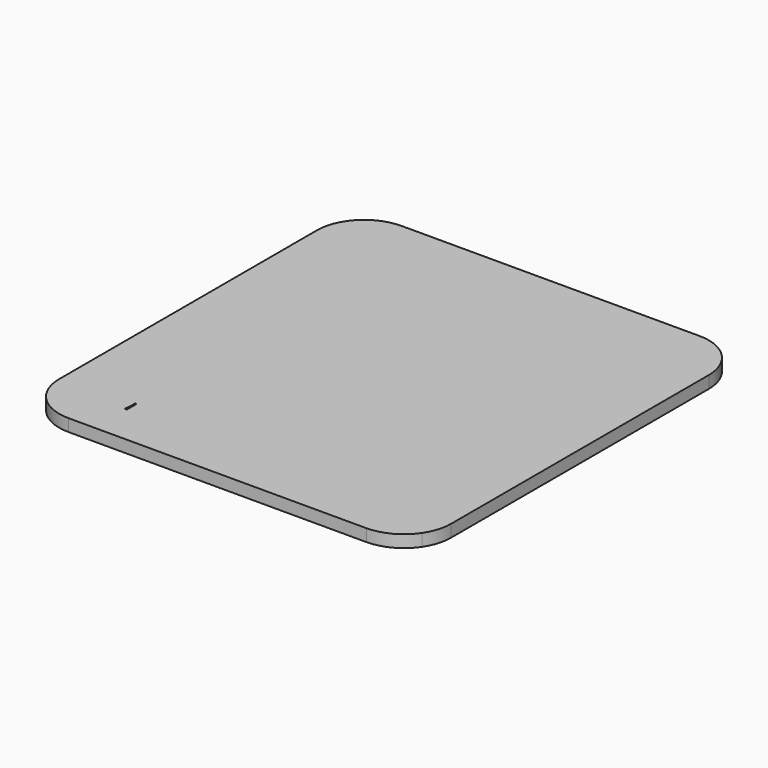
from build123d import *

# Parameters (mm, degrees)
F1_DEPTH = 2
F2_DEPTH = 2
F4_W     = 38
F4_H     = 4
F4_W_2   = 10
F5_DEPTH = 3


# Not quite as in the source:
# - a feature names something its author has since deleted; it is built from what else it names


with BuildPart() as f1:
    # F0 (on Top) → F1 (new body)
    with BuildSketch(Plane.XY):
        with BuildLine():
            Line((24.3022678875, 34), (-24.3022678875, 34))
            ThreePointArc((-24.3022678875, 34), (-29.745386464, 31.745386464), (-32, 26.3022678875))
            Line((-32, 26.3022678875), (-32, 15.1276998222))
            Line((-32, 15.1276998222), (-30.5, 15.1276998222))
            Line((-30.5, 15.1276998222), (-30.5, 21.3020170704))
            Line((-30.5, 21.3020170704), (30.5, 21.3020170704))
            Line((30.5, 21.3020170704), (30.5, 14.2477769405))
            Line((30.5, 14.2477769405), (32, 14.2477769405))
            Line((32, 14.2477769405), (32, 26.3022678875))
            ThreePointArc((32, 26.3022678875), (29.745386464, 31.745386464), (24.3022678875, 34))
        make_face()
        with BuildLine():
            Line((-30.5, 15.1276998222), (-32, 15.1276998222))
            Line((-32, 15.1276998222), (-32, -26.3022678875))
            ThreePointArc((-32, -26.3022678875), (-29.745386464, -31.745386464), (-24.3022678875, -34))
            Line((-24.3022678875, -34), (0, -34))
            Line((0, -34), (24.3022678875, -34))
            ThreePointArc((24.3022678875, -34), (27.9138443036, -33.100178998), (30.6810753302, -30.6110838832))
            ThreePointArc((30.6810753302, -30.6110838832), (31.6628871063, -28.555346757), (32, -26.3022678875))
            Line((32, -26.3022678875), (32, 14.2477769405))
            Line((32, 14.2477769405), (30.5, 14.2477769405))
            Line((30.5, 14.2477769405), (30.5, -14.6979829296))
            Line((30.5, -14.6979829296), (-30.5, -14.6979829296))
            Line((-30.5, -14.6979829296), (-30.5, 15.1276998222))
        make_face()
        with BuildLine():
            ThreePointArc((-20.3994758379, -27.4899639189), (-30.2031719041, -25.7844938681), (-20.255592559, -25.5261339915))
            Line((-20.255592559, -25.5261339915), (-20, -25.5261339915))
            Line((-20, -25.5261339915), (-20, -27.4899639189))
            Line((-20, -27.4899639189), (-20.3994758379, -27.4899639189))
        make_face(mode=Mode.SUBTRACT)
        with BuildLine():
            ThreePointArc((20.2726339823, -25.4029799253), (25.5910239568, -21.1638916046), (30.2165381279, -26.1498479185))
            ThreePointArc((30.2165381279, -26.1498479185), (25.7296627026, -31.1234485429), (20.3218568596, -27.1706786007))
            ThreePointArc((20.3218568596, -27.1706786007), (20.2184754644, -26.2890226707), (20.2726339823, -25.4029799253))
        make_face(mode=Mode.SUBTRACT)
        Polygon((-30.5, 21.3020170704), (-30.5, 15.1276998222), (-30.5, -14.6979829296), (30.5, -14.6979829296), (30.5, 14.2477769405), (30.5, 21.3020170704), align=None)
    extrude(amount=F1_DEPTH)

    # F0 (on Top) → F2 (join)
    with BuildSketch(Plane.XY):
        with BuildLine():
            ThreePointArc((-20.3994758379, -27.4899639189), (-20.2624836545, -26.8261202565), (-20.2165381279, -26.1498479185))
            ThreePointArc((-20.2165381279, -26.1498479185), (-20.2263112871, -25.8373801956), (-20.255592559, -25.5261339915))
            ThreePointArc((-20.255592559, -25.5261339915), (-30.2031719041, -25.7844938681), (-20.3994758379, -27.4899639189))
        make_face()
        with BuildLine():
            ThreePointArc((20.3218568596, -27.1706786007), (25.7296627026, -31.1234485429), (30.2165381279, -26.1498479185))
            ThreePointArc((30.2165381279, -26.1498479185), (25.5910239568, -21.1638916046), (20.2726339823, -25.4029799253))
            ThreePointArc((20.2726339823, -25.4029799253), (20.2184754644, -26.2890226707), (20.3218568596, -27.1706786007))
        make_face()
    extrude(amount=F2_DEPTH)

    # F4 (on face) → F5 (join)
    with BuildSketch(Plane.XY):
        with Locations((-0.7767596692, 27.0571730584)):
            Rectangle(F4_W, F4_H)
        with Locations((14.1091264039, -18.375430584)):
            Rectangle(F4_W_2, F4_H)
        with Locations((-14.1091264039, -18.375430584)):
            Rectangle(F4_W_2, F4_H)
    extrude(amount=-F5_DEPTH)


solid = f1.part
